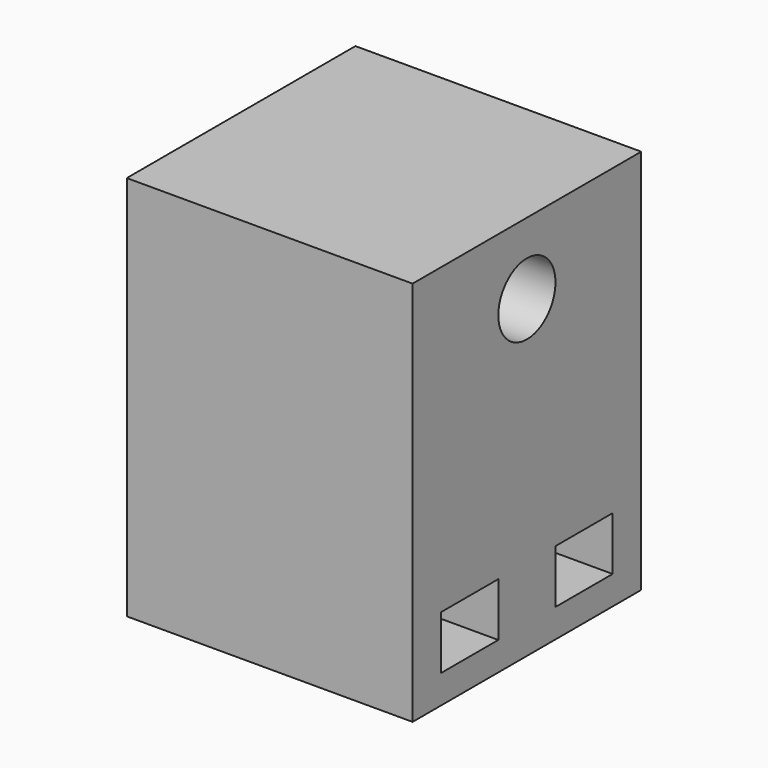
from build123d import *

# Parameters (mm, degrees)
F0_W     = 80
F0_H     = 80
F1_DEPTH = 50
F2_R     = 5
F3_DEPTH = 10
F4_R     = 10
F5_DEPTH = 86.1
F6_W     = 20
F6_H     = 15
F7_DEPTH = 84.6
F2_W     = 80
F2_H     = 80
F8_DEPTH = 8


# Not quite as in the source:
# - a pattern or mirror of a feature is missing from the dataset's text; its kind, count and spacing are read off the source's solid


with BuildPart() as f1:
    # F0 (on Top) → F1 (new body, symmetric)
    with BuildSketch(Plane.XY):
        Rectangle(F0_W, F0_H)
    extrude(amount=F1_DEPTH, both=True)

    # F2 (on face) → F3 (cut)
    with BuildSketch(Plane(origin=(0, 0, -50), x_dir=(1, 0, 0), z_dir=(0, 0, -1))):
        with Locations((-20, 20)):
            Circle(F2_R)
        with Locations((-20, -20)):
            Circle(F2_R)
        with Locations((20, -20)):
            Circle(F2_R)
        with Locations((20, 20)):
            Circle(F2_R)
    extrude(amount=-F3_DEPTH, mode=Mode.SUBTRACT)

    # F4 (on face) → F5 (cut)
    with BuildSketch(Plane(origin=(-40, 0, 0), x_dir=(0, -1, 0), z_dir=(-1, 0, 0))):
        with Locations((0, 30)):
            Circle(F4_R)
    extrude(amount=-F5_DEPTH, mode=Mode.SUBTRACT)

    # F6 (on face) → F7 (cut)
    with BuildSketch(Plane(origin=(-40, 0, 0), x_dir=(0, -1, 0), z_dir=(-1, 0, 0))):
        with Locations((-20, -42.5)):
            Rectangle(F6_W, F6_H)
    f7 = extrude(amount=-F7_DEPTH, mode=Mode.SUBTRACT)

    # F7_copies: F7 across plane
    add(f7.mirror(Plane(origin=(0, 0, 0), x_dir=(0, 0, -1), z_dir=(0, -1, 0))), mode=Mode.SUBTRACT)

    # F2 (on face) → F8 (join)
    with BuildSketch(Plane(origin=(0, 0, -50), x_dir=(1, 0, 0), z_dir=(0, 0, -1))):
        Rectangle(F2_W, F2_H)
        with Locations((-20, -20)):
            Circle(F2_R, mode=Mode.SUBTRACT)
        with Locations((20, -20)):
            Circle(F2_R, mode=Mode.SUBTRACT)
        with Locations((-20, 20)):
            Circle(F2_R, mode=Mode.SUBTRACT)
        with Locations((20, 20)):
            Circle(F2_R, mode=Mode.SUBTRACT)
    extrude(amount=F8_DEPTH)


solid = f1.part
